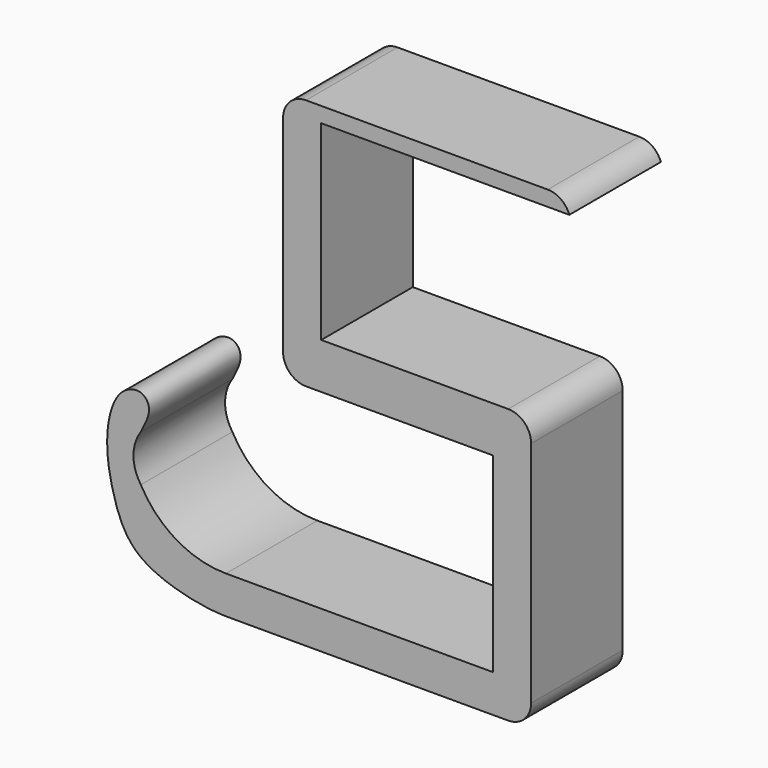
from build123d import *

# Parameters (mm, degrees)
F1_DEPTH    = 30
F2_T1_DEPTH = 60
F2_T3_DEPTH = 58.2842712475


# Not quite as in the source:
# - a fillet or chamfer that OpenCascade refuses, or shapes differently, is made with other operations: its cross-section is extruded or revolved along the edge and cut away or added


with BuildPart() as f1:
    # F0 (on Front) → F1 (new body)
    with BuildSketch(Plane.XZ):
        with BuildLine():
            Line((-20.4576485604, 41.7964319587), (44.5423514396, 41.7964319587))
            Line((44.5423514396, 41.7964319587), (44.5423514396, 45.7964319587))
            Line((44.5423514396, 45.7964319587), (-30.4576485604, 45.7964319587))
            Line((-30.4576485604, 45.7964319587), (-30.4576485604, -20.2035680413))
            Line((-30.4576485604, -20.2035680413), (24.5423514396, -20.2035680413))
            Line((24.5423514396, -20.2035680413), (24.5423514396, -70.2035680413))
            Line((24.5423514396, -70.2035680413), (-45.4576485604, -70.2035680413))
            ThreePointArc((-45.4576485604, -70.2035680413), (-58.4112677552, -66.6488561684), (-67.7362307906, -56.9804906845))
            ThreePointArc((-67.7362307906, -56.9804906845), (-69.6667608001, -50.8724953979), (-67.7362307906, -44.7645001113))
            add(Edge.make_bspline(
                [(-67.7362307906, -44.7645001113), (-66.6047282738, -42.6134626855), (-64.6275870644, -38.8548278844), (-67.5118728603, -34.7496923274), (-74.2171267591, -36.6728128022), (-77.5629423301, -48.422372807), (-75.1680740571, -62.4394566894), (-69.641186524, -75.442468141), (-51.6938526184, -79.943801044), (-46.7813036843, -80.045612986), (-44.8976382613, -80.0846517086)],
                knots=[0, 0, 0, 0, 0.1047159829, 0.1829764247, 0.2776975731, 0.4158396611, 0.5724266185, 0.7228497918, 0.8937296562, 1, 1, 1, 1], degree=3))
            Line((-44.8976382613, -80.0846517086), (34.5423514396, -80.0846517086))
            Line((34.5423514396, -80.0846517086), (34.5423514396, -8.2035680413))
            Line((34.5423514396, -8.2035680413), (-20.4576485604, -8.2035680413))
            Line((-20.4576485604, -8.2035680413), (-20.4576485604, 41.7964319587))
        make_face()
    extrude(amount=F1_DEPTH)

    # F2: fillet of radius 6 on 5 edges, made by hand

    # F2_s2 → F2_t1 (cut)
    with BuildSketch(Plane.XZ.offset(-15)):
        with BuildLine():
            ThreePointArc((-24.4576485604, 45.7964319587), (-28.7002892475, 44.0390726458), (-30.4576485604, 39.7964319587))
            Line((-30.4576485604, 39.7964319587), (-30.4576485604, 45.7964319587))
            Line((-30.4576485604, 45.7964319587), (-24.4576485604, 45.7964319587))
        make_face()
        with BuildLine():
            ThreePointArc((-30.4576485604, -14.2035680413), (-28.7002892475, -18.4462087284), (-24.4576485604, -20.2035680413))
            Line((-24.4576485604, -20.2035680413), (-30.4576485604, -20.2035680413))
            Line((-30.4576485604, -20.2035680413), (-30.4576485604, -14.2035680413))
        make_face()
        with BuildLine():
            ThreePointArc((34.5423514396, -14.2035680413), (32.7849921267, -9.9609273542), (28.5423514396, -8.2035680413))
            Line((28.5423514396, -8.2035680413), (34.5423514396, -8.2035680413))
            Line((34.5423514396, -8.2035680413), (34.5423514396, -14.2035680413))
        make_face()
        with BuildLine():
            ThreePointArc((28.5423514396, -80.0846517086), (32.7849921267, -78.3272923957), (34.5423514396, -74.0846517086))
            Line((34.5423514396, -74.0846517086), (34.5423514396, -80.0846517086))
            Line((34.5423514396, -80.0846517086), (28.5423514396, -80.0846517086))
        make_face()
    extrude(amount=F2_T1_DEPTH, mode=Mode.SUBTRACT)

    # F2_s4 → F2_t3 (cut)
    with BuildSketch(Plane.XZ.offset(-14.1421356237)):
        with BuildLine():
            ThreePointArc((44.5423514396, 41.7964319587), (42.3495988052, 44.6954114442), (38.8854971901, 45.7964319587))
            Line((38.8854971901, 45.7964319587), (44.5423514396, 45.7964319587))
            Line((44.5423514396, 45.7964319587), (44.5423514396, 41.7964319587))
        make_face()
    extrude(amount=F2_T3_DEPTH, mode=Mode.SUBTRACT)


solid = f1.part
